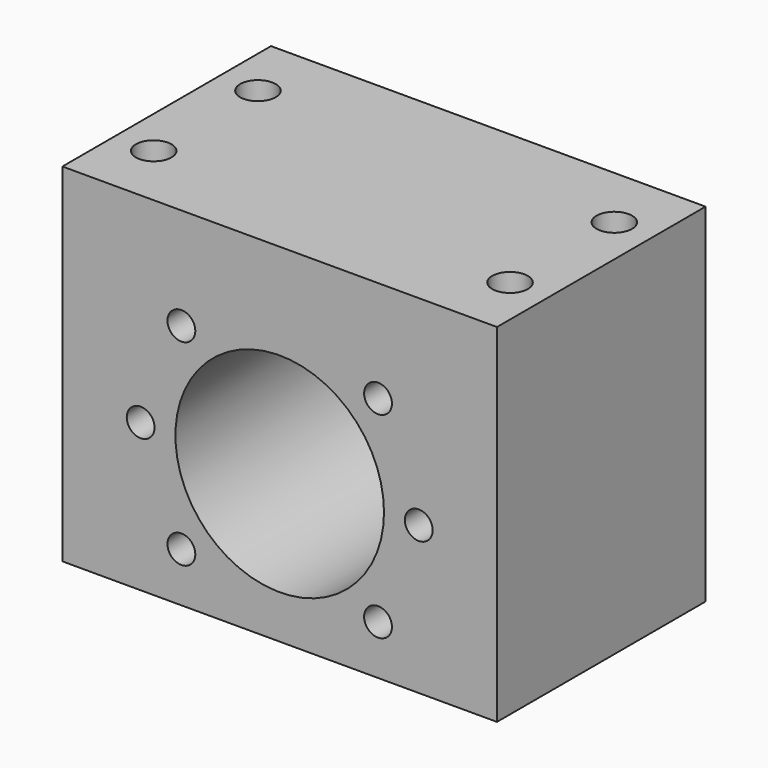
from build123d import *

# Parameters (mm, degrees)
F0_W     = 50
F0_H     = 40
F1_DEPTH = 30
F2_R     = 12
F3_DEPTH = 30.001
F4_D     = 3.2
F6_D     = 4.1


# Not quite as in the source:
# - a feature names something its author has since deleted; it is built from what else it names


with BuildPart() as f1:
    # F0 (on Front) → F1 (new body)
    with BuildSketch(Plane.XZ):
        with Locations((3.412880823, -1.3936108311)):
            Rectangle(F0_W, F0_H)
    extrude(amount=F1_DEPTH)

    # F2 (on face) → F3 (cut, through all)
    with BuildSketch(Plane.XZ.offset(30)):
        with Locations((3.412880823, -4.3936108311)):
            Circle(F2_R)
    extrude(amount=-F3_DEPTH, mode=Mode.SUBTRACT)

    # F4 (through all)
    with Locations(Plane.XZ.offset(30)):
        with Locations((-7.900827676, 6.9200976679), (-12.587119177, -4.3936108311), (-7.900827676, -15.7073193301), (14.726589322, -15.7073193301), (19.412880823, -4.3936108311), (14.726589322, 6.9200976679)):
            Hole(F4_D / 2)

    # F6 (through all)
    with Locations(Plane.XY.offset(18.6063891689)):
        with Locations((23.912880823, -22.5), (23.912880823, -7.5), (-17.087119177, -7.5), (-17.087119177, -22.5)):
            Hole(F6_D / 2)


solid = f1.part
